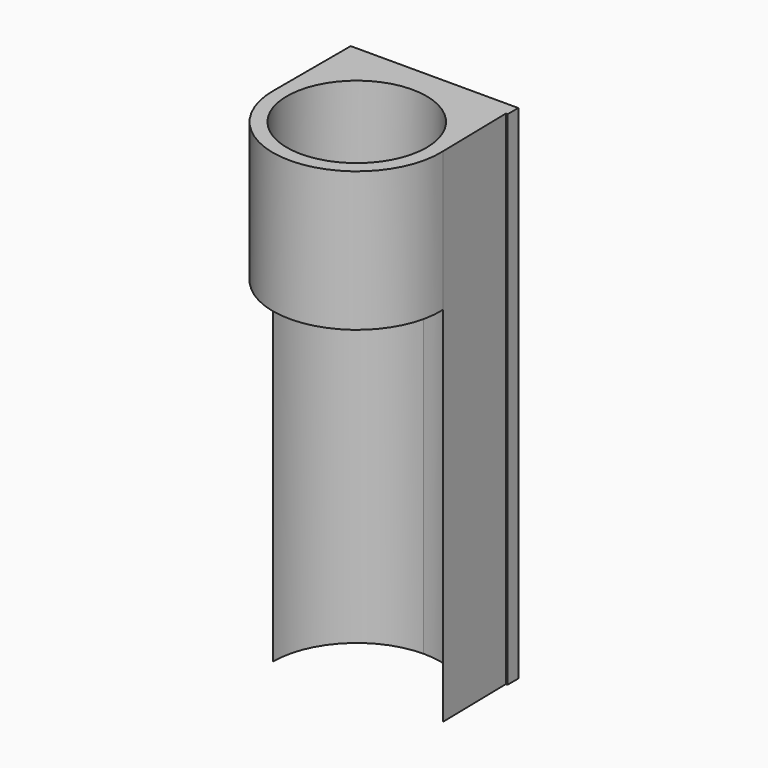
from build123d import *

# Parameters (mm, degrees)
F0_R     = 3.81
F0_R_2   = 3.175
F1_DEPTH = 6.35
F3_DEPTH = 22.86


with BuildPart() as f1:
    # F0 (on Top) → F1 (new body)
    with BuildSketch(Plane.XY):
        with Locations((0, -1.3826612849)):
            Circle(F0_R)
        with Locations((0, -1.3826612849)):
            Circle(F0_R_2, mode=Mode.SUBTRACT)
    extrude(amount=F1_DEPTH)

    # F2 (on face) → F3 (join)
    with BuildSketch(Plane.XY.offset(6.35)):
        with BuildLine():
            Line((-3.81, 2.4273387151), (-3.81, -1.3826612849))
            ThreePointArc((-3.81, -1.3826612849), (-2.6940768363, 1.3114155514), (0, 2.4273387151))
            Line((0, 2.4273387151), (-3.81, 2.4273387151))
        make_face()
        Polygon((-3.81, 2.4273387151), (0, 2.4273387151), (3.7383490708, 2.4273387151), (3.8155771326, 2.4273387151), (3.8155771326, 3.0369387151), (-3.81, 3.0369387151), align=None)
        with BuildLine():
            Line((3.7383490708, 2.4273387151), (0, 2.4273387151))
            ThreePointArc((0, 2.4273387151), (2.6429446594, 1.3615951767), (3.8073060154, -1.2394100895))
            Line((3.8073060154, -1.2394100895), (3.7383490708, 2.4273387151))
        make_face()
    extrude(amount=-F3_DEPTH)


solid = f1.part
